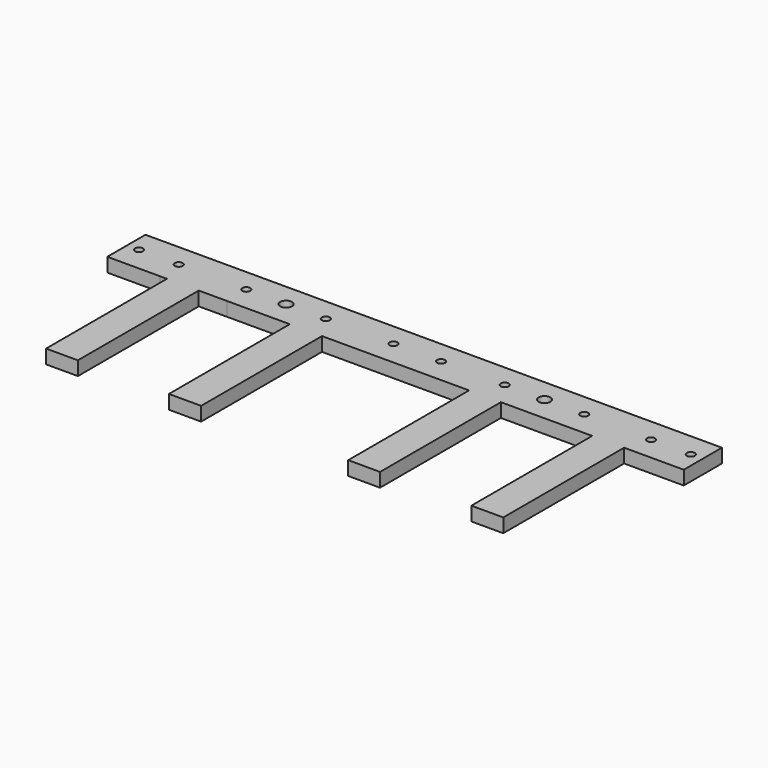
from build123d import *

# Parameters (mm, degrees)
F0_W     = 2.9513968527
F0_H     = 5.7922647223
F0_W_2   = 10.2618969977
F0_H_2   = 6.2077352777
F0_W_3   = 16.8588273227
F0_W_4   = 37.1382929152
F0_W_5   = 8
F0_H_3   = 38
F0_W_6   = 8.1014430672
F0_W_7   = 8.0087523311
F0_W_8   = 8.027805835
F1_DEPTH = 3.5
F2_D     = 2
F3_D     = 3


# Not quite as in the source:
# - a feature names something its author has since deleted; it is built from what else it names


with BuildPart() as f1:
    # F0 (on Top) → F1 (new body)
    with BuildSketch(Plane.XY):
        with Locations((-67.6180190593, 24.675444182)):
            Rectangle(F0_W, F0_H)
        with Locations((-61.0113721341, 24.675444182)):
            Rectangle(F0_W_2, F0_H)
        with Locations((-67.6180190593, 18.675444182)):
            Rectangle(F0_W, F0_H_2)
        with Locations((-47.4510099739, 24.675444182)):
            Rectangle(F0_W_3, F0_H)
        with Locations((-61.0113721341, 18.675444182)):
            Rectangle(F0_W_2, F0_H_2)
        with Locations((-20.4524498549, 24.675444182)):
            Rectangle(F0_W_4, F0_H)
        Polygon((-39.0215963125, 21.7793118209), (-55.8804236352, 21.7793118209), (-55.8804236352, 15.5715765432), (-54.0937174857, 15.5715765432), (-46.0937174857, 15.5715765432), (-39.0215963125, 15.5715765432), align=None)
        Polygon((9.8445750773, 27.5715765432), (-1.8833033973, 27.5715765432), (-1.8833033973, 21.7793118209), (9.8743605615, 21.7793118209), align=None)
        Polygon((-1.8833033973, 21.7793118209), (-39.0215963125, 21.7793118209), (-39.0215963125, 15.5715765432), (-23.1951605529, 15.5715765432), (-15.0937174857, 15.5715765432), (-1.8833033973, 15.5715765432), align=None)
        Polygon((62.8643706441, 27.5715765432), (9.8445750773, 27.5715765432), (9.8743605615, 21.7793118209), (62.8643706441, 21.7793118209), align=None)
        Polygon((9.8743605615, 21.7793118209), (-1.8833033973, 21.7793118209), (-1.8833033973, 15.5715765432), (9.9062825143, 15.5715765432), align=None)
        with Locations((-50.0937174857, -3.4284234568)):
            Rectangle(F0_W_5, F0_H_3)
        Polygon((72.6376026869, 27.5715765432), (62.8643706441, 27.5715765432), (62.8643706441, 21.7793118209), (72.7672914107, 21.7793118209), align=None)
        Polygon((62.8643706441, 21.7793118209), (9.8743605615, 21.7793118209), (9.9062825143, 15.5715765432), (21.8975301832, 15.5715765432), (29.9062825143, 15.5715765432), (52.8784766793, 15.5715765432), (60.9062825143, 15.5715765432), (62.8643706441, 15.5715765432), align=None)
        with Locations((-19.1444390193, -3.4284234568)):
            Rectangle(F0_W_6, F0_H_3)
        Polygon((75.9062825143, 27.5715765432), (72.6376026869, 27.5715765432), (72.7672914107, 21.7793118209), (75.9062825143, 21.7793118209), align=None)
        Polygon((72.7672914107, 21.7793118209), (62.8643706441, 21.7793118209), (62.8643706441, 15.5715765432), (72.9062825143, 15.5715765432), align=None)
        Polygon((75.9062825143, 21.7793118209), (72.7672914107, 21.7793118209), (72.9062825143, 15.5715765432), (75.9062825143, 15.5715765432), align=None)
        with Locations((25.9019063488, -3.4284234568)):
            Rectangle(F0_W_7, F0_H_3)
        with Locations((56.8923795968, -3.4284234568)):
            Rectangle(F0_W_8, F0_H_3)
    extrude(amount=F1_DEPTH)

    # F2 (through all)
    with Locations(Plane(origin=(0, 0, 0), x_dir=(1, 0, 0), z_dir=(0, 0, -1))):
        with Locations((-66.0937174857, -21.7793118209), (-56.0937174857, -21.7793118209), (-39.0937174857, -21.7793118209), (-19.0937174857, -21.7793118209), (-2.0937174857, -21.7793118209), (9.9062825143, -21.7793118209), (25.9062825143, -21.7793118209), (45.9062825143, -21.7793118209), (62.9062825143, -21.5349812061), (72.9062825143, -21.5349812061)):
            Hole(F2_D / 2)

    # F3 (through all)
    with Locations(Plane(origin=(0, 0, 0), x_dir=(1, 0, 0), z_dir=(0, 0, -1))):
        with Locations((-29.0937174857, -21.7793118209), (35.9062825143, -21.7793118209)):
            Hole(F3_D / 2)


solid = f1.part
